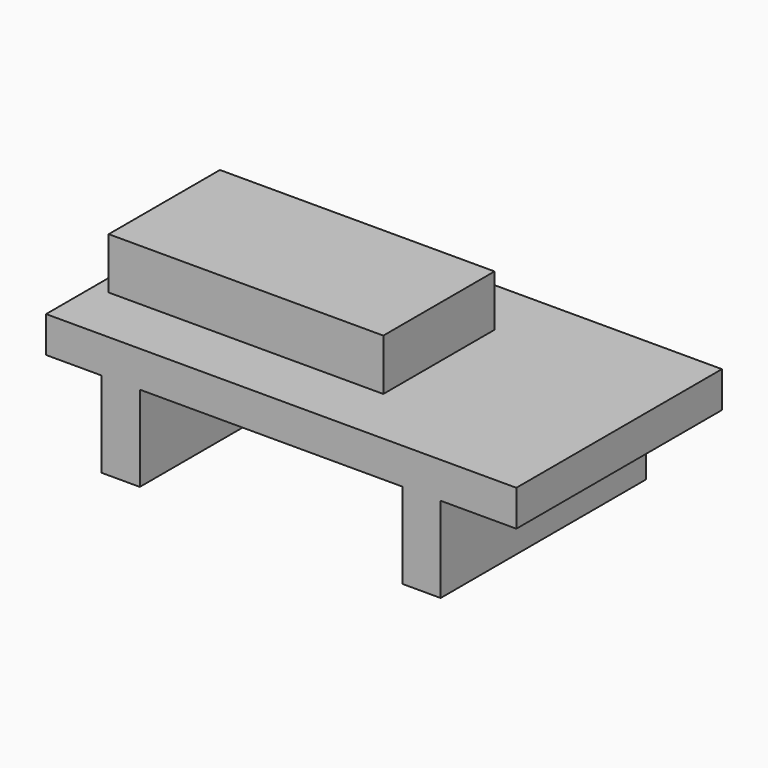
from build123d import *

# Parameters (mm, degrees)
F0_W     = 139.4626796246
F0_H     = 10.6887500733
F1_DEPTH = 38.1
F2_W     = 139.4626796246
F2_H     = 10.6887500733
F3_DEPTH = 38.1
F4_W     = 11.3281075606
F4_H     = 76.2
F5_DEPTH = 25.4
F6_W     = 11.3281150824
F6_H     = 76.2
F7_DEPTH = 25.4
F8_W     = 81.4380571246
F8_H     = 41.2280112505
F9_DEPTH = 15.24


# Not quite as in the source:
# - the program builds the solid bodies; features that only make, move or delete a surface that nothing else refers to are left out


with BuildPart() as f1:
    # F0 (on Front) → F1 (new body)
    with BuildSketch(Plane.XZ):
        Rectangle(F0_W, F0_H)
    extrude(amount=F1_DEPTH)

    # F2 (on face) → F3 (join)
    with BuildSketch(Plane(origin=(0, 0, 0), x_dir=(-1, 0, 0), z_dir=(0, 1, 0))):
        Rectangle(F2_W, F2_H)
    extrude(amount=F3_DEPTH)

    # F4 (on face) → F5 (join)
    with BuildSketch(Plane(origin=(0, 0, -5.3443750367), x_dir=(1, 0, 0), z_dir=(0, 0, -1))):
        with Locations((-47.5903637707, 0)):
            Rectangle(F4_W, F4_H)
    extrude(amount=F5_DEPTH)

    # F6 (on face) → F7 (join)
    with BuildSketch(Plane(origin=(0, 0, -5.3443750367), x_dir=(1, 0, 0), z_dir=(0, 0, -1))):
        with Locations((41.6097603738, 0)):
            Rectangle(F6_W, F6_H)
    extrude(amount=F7_DEPTH)

    # F8 (on face) → F9 (join)
    with BuildSketch(Plane.XY.offset(5.3443750367)):
        with Locations((-24.4314149022, 0)):
            Rectangle(F8_W, F8_H)
    extrude(amount=F9_DEPTH)


solid = f1.part
